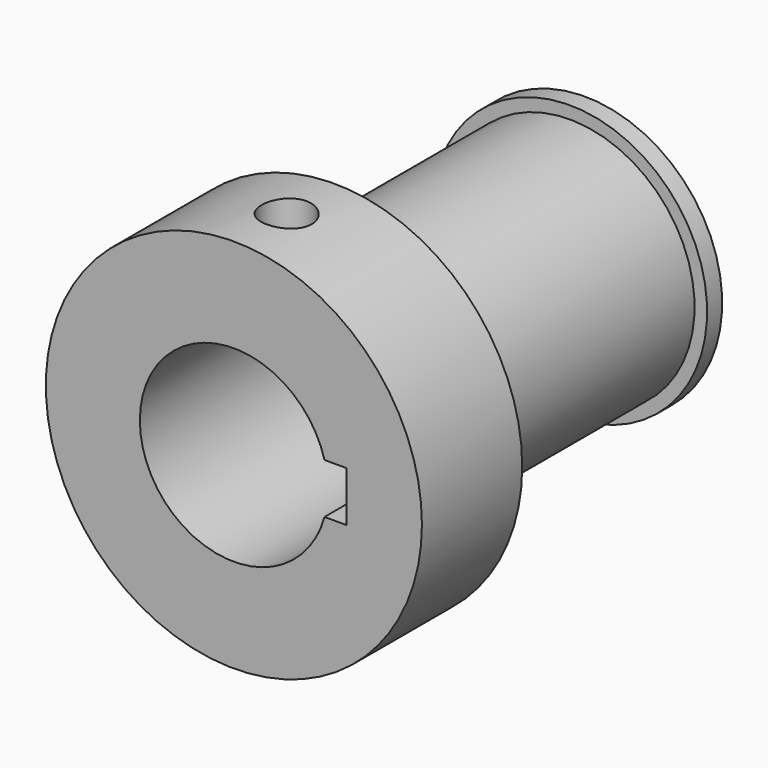
from build123d import *

# Parameters (mm, degrees)
F0_R      = 30
F1_DEPTH  = 20
F2_R      = 21.9
F3_DEPTH  = 5
F4_SIZE   = 2
F5_DEPTH  = 42
F6_R      = 21.9
F6_R_2    = 19.9
F7_DEPTH  = 3
F9_DEPTH  = 74.3
F11_R     = 4
F12_DEPTH = 25


with BuildPart() as f1:
    # F0 (on Front) → F1 (new body)
    with BuildSketch(Plane.XZ):
        with Locations((61.7417618632, 67.357480526)):
            Circle(F0_R)
    extrude(amount=F1_DEPTH)

    # F2 (on face) → F3 (join)
    with BuildSketch(Plane(origin=(0, 0, 0), x_dir=(-1, 0, 0), z_dir=(0, 1, 0))):
        with Locations((-61.7417618632, 67.357480526)):
            Circle(F2_R)
    extrude(amount=F3_DEPTH)

    # F4
    f4_edges = [f1.edges().sort_by_distance(p)[0] for p in [
        (83.641762, 5, 67.357481),
    ]]
    chamfer(f4_edges, length=F4_SIZE)

    # F5 (add): a face of the model
    f5_faces = [f1.faces().sort_by_distance(p)[0] for p in [
        (61.7417618632, 5, 67.357480526),
    ]]
    extrude(f5_faces, amount=F5_DEPTH)

    # F6 (on face) → F7 (join)
    with BuildSketch(Plane(origin=(0, 47, 0), x_dir=(-1, 0, 0), z_dir=(0, 1, 0))):
        with Locations((-61.7417618632, 67.357480526)):
            Circle(F6_R)
        with Locations((-61.7417618632, 67.357480526)):
            Circle(F6_R_2, mode=Mode.SUBTRACT)
        with Locations((-61.7417618632, 67.357480526)):
            Circle(F6_R_2)
    extrude(amount=F7_DEPTH)

    # F8 (on face) → F9 (cut)
    with BuildSketch(Plane(origin=(0, 50, 0), x_dir=(-1, 0, 0), z_dir=(0, 1, 0))):
        with BuildLine():
            Line((-79.7417618632, 63.357480526), (-76.198594158, 63.357480526))
            ThreePointArc((-76.198594158, 63.357480526), (-46.7417618632, 67.357480526), (-76.198594158, 71.357480526))
            Line((-76.198594158, 71.357480526), (-79.7417618632, 71.357480526))
            Line((-79.7417618632, 71.357480526), (-79.7417618632, 67.357480526))
            Line((-79.7417618632, 67.357480526), (-79.7417618632, 63.357480526))
        make_face()
    extrude(amount=-F9_DEPTH, mode=Mode.SUBTRACT)

    # F11 (on offset) → F12 (cut)
    with BuildSketch(Plane.XY.offset(100)):
        with Locations((62.0413188264, -9.8582830757)):
            Circle(F11_R)
    extrude(amount=-F12_DEPTH, mode=Mode.SUBTRACT)


solid = f1.part
